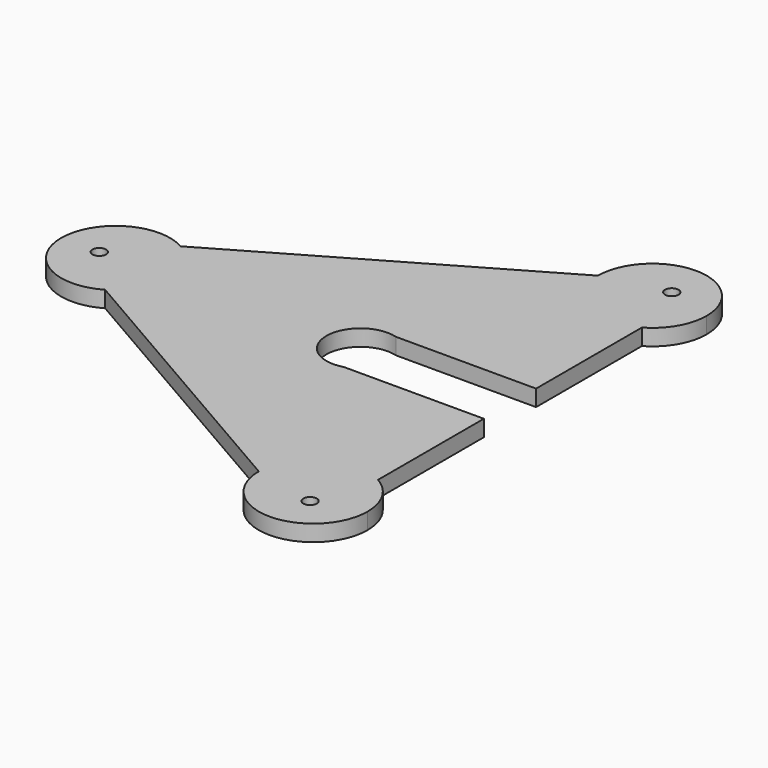
from build123d import *

# Parameters (mm, degrees)
F1_DEPTH        = 6
F2_R            = 12.5
F3_DEPTH        = 6
F4_R            = 2.5
F5_DEPTH        = 6
F5_COPIES_COUNT = 3
F6_W            = 60
F6_H            = 24
F7_DEPTH        = 6


# Not quite as in the source:
# - a pattern or mirror of a feature is missing from the dataset's text; its kind, count and spacing are read off the source's solid


with BuildPart() as f1:
    # F0 (on Top) → F1 (new body)
    with BuildSketch(Plane.XY):
        with BuildLine():
            ThreePointArc((-80, 17.3205080757), (-100, 17.3205080757), (-110, 0))
            Line((-110, 0), (-80, 17.3205080757))
        make_face()
        with BuildLine():
            Line((-80, 17.3205080757), (-110, 0))
            Line((-110, 0), (-80, -17.3205080757))
            ThreePointArc((-80, -17.3205080757), (-72.6794919243, -10), (-70, 0))
            ThreePointArc((-70, 0), (-72.6794919243, 10), (-80, 17.3205080757))
        make_face()
        with BuildLine():
            Line((-80, -17.3205080757), (-110, 0))
            ThreePointArc((-110, 0), (-100, -17.3205080757), (-80, -17.3205080757))
        make_face()
        with BuildLine():
            Line((25, 77.9422863406), (-80, 17.3205080757))
            ThreePointArc((-80, 17.3205080757), (-72.6794919243, 10), (-70, 0))
            ThreePointArc((-70, 0), (-72.6794919243, -10), (-80, -17.3205080757))
            Line((-80, -17.3205080757), (25, -77.9422863406))
            ThreePointArc((25, -77.9422863406), (35, -60.6217782649), (55, -60.6217782649))
            Line((55, -60.6217782649), (55, 60.6217782649))
            ThreePointArc((55, 60.6217782649), (35, 60.6217782649), (25, 77.9422863406))
        make_face()
        with BuildLine():
            ThreePointArc((55, 95.2627944163), (35, 95.2627944163), (25, 77.9422863406))
            Line((25, 77.9422863406), (55, 95.2627944163))
        make_face()
        with BuildLine():
            Line((55, 95.2627944163), (25, 77.9422863406))
            ThreePointArc((25, 77.9422863406), (35, 60.6217782649), (55, 60.6217782649))
            Line((55, 60.6217782649), (55, 95.2627944163))
        make_face()
        with BuildLine():
            ThreePointArc((55, -60.6217782649), (35, -60.6217782649), (25, -77.9422863406))
            Line((25, -77.9422863406), (55, -95.2627944163))
            Line((55, -95.2627944163), (55, -60.6217782649))
        make_face()
        with BuildLine():
            Line((55, -95.2627944163), (25, -77.9422863406))
            ThreePointArc((25, -77.9422863406), (35, -95.2627944163), (55, -95.2627944163))
        make_face()
        with BuildLine():
            ThreePointArc((65, 77.9422863406), (62.3205080757, 87.9422863406), (55, 95.2627944163))
            Line((55, 95.2627944163), (55, 60.6217782649))
            ThreePointArc((55, 60.6217782649), (62.3205080757, 67.9422863406), (65, 77.9422863406))
        make_face()
        with BuildLine():
            Line((55, -60.6217782649), (55, -95.2627944163))
            ThreePointArc((55, -95.2627944163), (62.3205080757, -87.9422863406), (65, -77.9422863406))
            ThreePointArc((65, -77.9422863406), (62.3205080757, -67.9422863406), (55, -60.6217782649))
        make_face()
    extrude(amount=F1_DEPTH)

    # F2 (on face) → F3 (cut, through all)
    with BuildSketch(Plane.XY.offset(6)):
        Circle(F2_R)
    extrude(amount=-F3_DEPTH, mode=Mode.SUBTRACT)

    # F4 (on face) → F5 (cut, through all)
    with BuildSketch(Plane.XY.offset(6)):
        with Locations((-96, 0)):
            Circle(F4_R)
    f5 = extrude(amount=-F5_DEPTH, mode=Mode.SUBTRACT)

    # F5_copies: F5 ×3 about axis
    f5_copies_axis = Axis((0, 0, 0), (0, 0, 1))
    for i in range(1, F5_COPIES_COUNT):
        add(f5.rotate(f5_copies_axis, i * 360 / F5_COPIES_COUNT), mode=Mode.SUBTRACT)

    # F6 (on face) → F7 (cut, through all)
    with BuildSketch(Plane.XY.offset(6)):
        with Locations((33.5, 0)):
            Rectangle(F6_W, F6_H)
    extrude(amount=-F7_DEPTH, mode=Mode.SUBTRACT)


solid = f1.part
